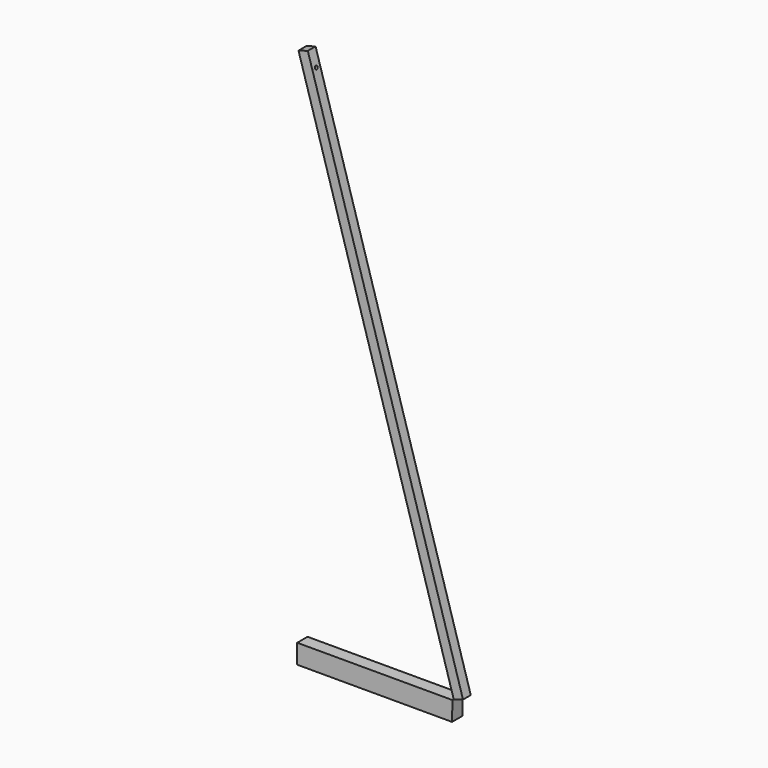
from build123d import *

# Parameters (mm, degrees)
F1_DEPTH = 19.05
F3_D     = 12.7
F3_DEPTH = 609.6
F3_START = 505.845639
F3_TIP   = 3.815465
F4_DEPTH = 25.4
F7_D     = 0.254
F7_DEPTH = 598.320788


with BuildPart() as f1:
    # F0 (on Front) → F1 (new body, symmetric)
    with BuildSketch(Plane.XZ):
        Polygon((-503.736335, 1056.839082), (-543.493624, 1056.839082), (51.209012, -937.854198), (87.720808, -926.968484), align=None)
        Polygon((-521.879192, 1117.692075), (-558.390988, 1106.80636), (-543.493624, 1056.839082), (-503.736335, 1056.839082), align=None)
    extrude(amount=F1_DEPTH, both=True)

    # F3
    # its depths count from where the whole tool has entered the part; down to there all is cleared
    with Locations(Plane.YZ.offset(-F3_START)):
        with Locations((0, 1057.563901)):
            Hole(F3_D / 2, depth=F3_DEPTH)
            with Locations((0, 0, -(F3_DEPTH + F3_TIP / 2))):  # 118° drill point
                Cone(0, F3_D / 2, F3_TIP, mode=Mode.SUBTRACT)

    # F7 (through all, one way)
    with BuildSketch(Plane.YZ.offset(39.9288)):
        with Locations((0, -899.086475)):
            Circle(F7_D / 2)
    extrude(amount=-F7_DEPTH, mode=Mode.SUBTRACT)


with BuildPart() as f4:
    # F0 (on Front) → F4 (new body, symmetric)
    with BuildSketch(Plane.XZ):
        Polygon((51.209012, -937.854198), (-558.390988, -937.854198), (-558.390988, -1013.908505), (49.638357, -1013.908505), align=None)
    extrude(amount=F4_DEPTH, both=True)


solid = Compound([f1.part, f4.part])
